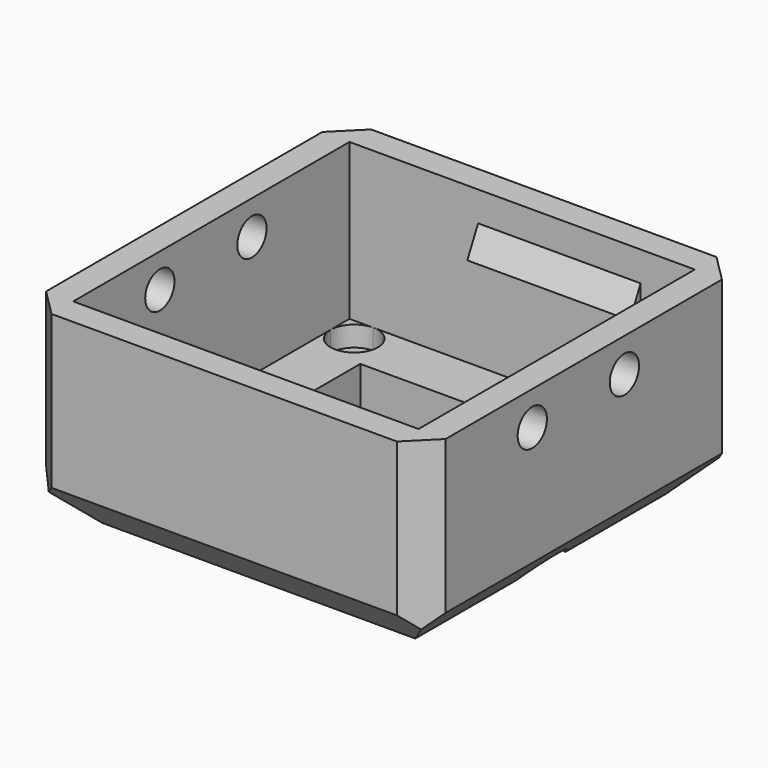
from build123d import *

# Parameters (mm, degrees)
F1_DEPTH     = 3
F0_W         = 29.5
F0_H         = 29.5
F2_DEPTH     = 14.5
F3_DEPTH     = 3
F4_DEPTH     = 1.5
F6_W         = 12
F6_H         = 2
F7_DEPTH     = 1
F8_SIZE2     = 1.99999
F8_SIZE      = 0.99999
F9_W         = 1.2
F9_H         = 2
F10_DEPTH    = 1
F11_SIZE2    = 1.99999
F11_SIZE     = 0.99999
F12_SIZE2    = 1.99999
F12_SIZE     = 0.99999
F13_T1_DEPTH = 45.958771123
F13_T3_DEPTH = 45.958771123
F5_R         = 1.35
F14_DEPTH    = 30
F15_SIZE     = 2


# Not quite as in the source:
# - a fillet or chamfer that OpenCascade refuses, or shapes differently, is made with other operations: its cross-section is extruded or revolved along the edge and cut away or added
# - a fillet or chamfer is up to 0.001 mm smaller than in the source, because OpenCascade refuses the exact size


with BuildPart() as f1:
    # F0 (on Top) → F1 (new body)
    with BuildSketch(Plane.XY):
        with BuildLine():
            ThreePointArc((12.75, 11), (9.7625631329, 9.7625631329), (11, 12.75))
            Line((11, 12.75), (-11, 12.75))
            ThreePointArc((-11, 12.75), (-9.7625631329, 12.2374368671), (-9.25, 11))
            ThreePointArc((-9.25, 11), (-11, 9.25), (-12.75, 11))
            Line((-12.75, 11), (-12.75, -5e-10))
            ThreePointArc((-12.75, -5e-10), (-11.9445436484, 1.9445436481), (-10, 2.75))
            Line((-10, 2.75), (-8.75, 2.75))
            Line((-8.75, 2.75), (-8.75, 8.75))
            Line((-8.75, 8.75), (8.75, 8.75))
            Line((8.75, 8.75), (8.75, 2.75))
            Line((8.75, 2.75), (10, 2.75))
            ThreePointArc((10, 2.75), (11.9445436484, 1.9445436481), (12.75, -5e-10))
            Line((12.75, -5e-10), (12.75, 11))
        make_face()
        with BuildLine():
            ThreePointArc((-12.75, 11), (-12.2374368671, 12.2374368671), (-11, 12.75))
            Line((-11, 12.75), (-12.75, 12.75))
            Line((-12.75, 12.75), (-12.75, 11))
        make_face()
        with BuildLine():
            Line((12.75, 11), (12.75, 12.75))
            Line((12.75, 12.75), (11, 12.75))
            ThreePointArc((11, 12.75), (12.2374368671, 12.2374368671), (12.75, 11))
        make_face()
        with BuildLine():
            ThreePointArc((12.75, 11), (12.2374368671, 12.2374368671), (11, 12.75))
            ThreePointArc((11, 12.75), (9.7625631329, 9.7625631329), (12.75, 11))
        make_face()
        with BuildLine():
            ThreePointArc((-9.25, 11), (-9.7625631329, 12.2374368671), (-11, 12.75))
            ThreePointArc((-11, 12.75), (-12.2374368671, 12.2374368671), (-12.75, 11))
            ThreePointArc((-12.75, 11), (-11, 9.25), (-9.25, 11))
        make_face()
    extrude(amount=F1_DEPTH)



with BuildPart() as f1b:
    # F0 (on Top) → F1, piece 2 (new body)
    with BuildSketch(Plane.XY):
        with BuildLine():
            Line((12.75, -11), (12.75, -5e-10))
            ThreePointArc((12.75, -5e-10), (11.9445436481, -1.9445436484), (10, -2.75))
            Line((10, -2.75), (8.75, -2.75))
            Line((8.75, -2.75), (8.75, -8.75))
            Line((8.75, -8.75), (-8.75, -8.75))
            Line((-8.75, -8.75), (-8.75, -2.75))
            Line((-8.75, -2.75), (-10, -2.75))
            ThreePointArc((-10, -2.75), (-11.9445436481, -1.9445436484), (-12.75, -5e-10))
            Line((-12.75, -5e-10), (-12.75, -11))
            ThreePointArc((-12.75, -11), (-11, -9.25), (-9.25, -11))
            ThreePointArc((-9.25, -11), (-9.7625631329, -12.2374368671), (-11, -12.75))
            Line((-11, -12.75), (11, -12.75))
            ThreePointArc((11, -12.75), (9.7625631329, -9.7625631329), (12.75, -11))
        make_face()
        with BuildLine():
            ThreePointArc((-11, -12.75), (-12.2374368671, -12.2374368671), (-12.75, -11))
            Line((-12.75, -11), (-12.75, -12.75))
            Line((-12.75, -12.75), (-11, -12.75))
        make_face()
        with BuildLine():
            Line((12.75, -12.75), (12.75, -11))
            ThreePointArc((12.75, -11), (12.2374368671, -12.2374368671), (11, -12.75))
            Line((11, -12.75), (12.75, -12.75))
        make_face()
        with BuildLine():
            ThreePointArc((11, -12.75), (12.2374368671, -12.2374368671), (12.75, -11))
            ThreePointArc((12.75, -11), (9.7625631329, -9.7625631329), (11, -12.75))
        make_face()
        with BuildLine():
            ThreePointArc((-9.25, -11), (-11, -9.25), (-12.75, -11))
            ThreePointArc((-12.75, -11), (-12.2374368671, -12.2374368671), (-11, -12.75))
            ThreePointArc((-11, -12.75), (-9.7625631329, -12.2374368671), (-9.25, -11))
        make_face()
    extrude(amount=F1_DEPTH)


with BuildPart() as f1_1:
    add(f1.part)

    add(f1b.part)  # F2 merges F1b
    # F0 (on Top) → F2 (join)
    with BuildSketch(Plane.XY):
        Rectangle(F0_W, F0_H)
        Polygon((11, 12.75), (12.75, 12.75), (12.75, 11), (12.75, -5e-10), (12.75, -11), (12.75, -12.75), (11, -12.75), (-11, -12.75), (-12.75, -12.75), (-12.75, -11), (-12.75, -5e-10), (-12.75, 11), (-12.75, 12.75), (-11, 12.75), align=None, mode=Mode.SUBTRACT)
    extrude(amount=F2_DEPTH)

    # F0 (on Top) → F3 (cut)
    with BuildSketch(Plane.XY):
        with BuildLine():
            ThreePointArc((-9.25, 11), (-9.7625631329, 12.2374368671), (-11, 12.75))
            ThreePointArc((-11, 12.75), (-12.2374368671, 12.2374368671), (-12.75, 11))
            ThreePointArc((-12.75, 11), (-11, 9.25), (-9.25, 11))
        make_face()
        with BuildLine():
            ThreePointArc((12.75, 11), (12.2374368671, 12.2374368671), (11, 12.75))
            ThreePointArc((11, 12.75), (9.7625631329, 9.7625631329), (12.75, 11))
        make_face()
        with BuildLine():
            ThreePointArc((-9.25, -11), (-11, -9.25), (-12.75, -11))
            ThreePointArc((-12.75, -11), (-12.2374368671, -12.2374368671), (-11, -12.75))
            ThreePointArc((-11, -12.75), (-9.7625631329, -12.2374368671), (-9.25, -11))
        make_face()
        with BuildLine():
            ThreePointArc((11, -12.75), (12.2374368671, -12.2374368671), (12.75, -11))
            ThreePointArc((12.75, -11), (9.7625631329, -9.7625631329), (11, -12.75))
        make_face()
    extrude(amount=F3_DEPTH, mode=Mode.SUBTRACT)

    # F0 (on Top) → F4 (join)
    with BuildSketch(Plane.XY):
        with BuildLine():
            ThreePointArc((12.75, 11), (12.2374368671, 12.2374368671), (11, 12.75))
            ThreePointArc((11, 12.75), (9.7625631329, 9.7625631329), (12.75, 11))
        make_face()
        with BuildLine():
            ThreePointArc((-9.25, 11), (-9.7625631329, 12.2374368671), (-11, 12.75))
            ThreePointArc((-11, 12.75), (-12.2374368671, 12.2374368671), (-12.75, 11))
            ThreePointArc((-12.75, 11), (-11, 9.25), (-9.25, 11))
        make_face()
        with BuildLine():
            ThreePointArc((-9.25, -11), (-11, -9.25), (-12.75, -11))
            ThreePointArc((-12.75, -11), (-12.2374368671, -12.2374368671), (-11, -12.75))
            ThreePointArc((-11, -12.75), (-9.7625631329, -12.2374368671), (-9.25, -11))
        make_face()
        with BuildLine():
            ThreePointArc((11, -12.75), (12.2374368671, -12.2374368671), (12.75, -11))
            ThreePointArc((12.75, -11), (9.7625631329, -9.7625631329), (11, -12.75))
        make_face()
    extrude(amount=F4_DEPTH)

    # F6 (on face) → F7 (join)
    with BuildSketch(Plane.XZ.offset(-12.75)):
        with Locations((2.75, 11.3)):
            Rectangle(F6_W, F6_H)
    extrude(amount=F7_DEPTH)

    # F8 (size 1 and 2 in the source; OpenCascade refuses exactly that, so slightly less here)
    f8_edges = [f1_1.edges().sort_by_distance(p)[0] for p in [
        (2.75, 11.75, 12.3),
    ]]
    f8_side = f1_1.faces().sort_by_distance((2.75, 12.25, 12.3))[0]
    chamfer(f8_edges, length=F8_SIZE, length2=F8_SIZE2, reference=f8_side)

    # F9 (on face) → F10 (join)
    with BuildSketch(Plane(origin=(0, -12.75, 0), x_dir=(-1, 0, 0), z_dir=(0, 1, 0))):
        with Locations((-8.85, 11.3)):
            Rectangle(F9_W, F9_H)
        with Locations((8.85, 11.3)):
            Rectangle(F9_W, F9_H)
    extrude(amount=F10_DEPTH)

    # F11 (size 1 and 2 in the source; OpenCascade refuses exactly that, so slightly less here)
    f11_edges = [f1_1.edges().sort_by_distance(p)[0] for p in [
        (8.85, -11.75, 12.3),
    ]]
    f11_side = f1_1.faces().sort_by_distance((8.85, -12.25, 12.3))[0]
    chamfer(f11_edges, length=F11_SIZE, length2=F11_SIZE2, reference=f11_side)

    # F12 (size 1 and 2 in the source; OpenCascade refuses exactly that, so slightly less here)
    f12_edges = [f1_1.edges().sort_by_distance(p)[0] for p in [
        (-8.85, -11.75, 12.3),
    ]]
    f12_side = f1_1.faces().sort_by_distance((-8.85, -12.25, 12.3))[0]
    chamfer(f12_edges, length=F12_SIZE, length2=F12_SIZE2, reference=f12_side)

    # F13: chamfer of 3.2 on 4 edges, made by hand

    # F13_s2 → F13_t1 (cut)
    with BuildSketch(Plane.YZ.offset(-22.9793855615)):
        Polygon((14.75, 3.2), (11.55, 0), (14.75, 0), align=None)
        Polygon((-14.75, 3.2), (-11.55, 0), (-14.75, 0), align=None)
    extrude(amount=F13_T1_DEPTH, mode=Mode.SUBTRACT)

    # F13_s4 → F13_t3 (cut)
    with BuildSketch(Plane.XZ.offset(-22.9793855615)):
        Polygon((-14.75, 3.2), (-11.55, 0), (-14.75, 0), align=None)
        Polygon((14.75, 3.2), (11.55, 0), (14.75, 0), align=None)
    extrude(amount=F13_T3_DEPTH, mode=Mode.SUBTRACT)

    # F5 (on face) → F14 (cut)
    with BuildSketch(Plane(origin=(-14.75, 0, 0), x_dir=(0, -1, 0), z_dir=(-1, 0, 0))):
        with Locations((4.75, 12)):
            Circle(F5_R)
        with Locations((-3.75, 12)):
            Circle(F5_R)
    extrude(amount=-F14_DEPTH, mode=Mode.SUBTRACT)

    # F15
    f15_edges = [f1_1.edges().sort_by_distance(p)[0] for p in [
        (14.75, 14.75, 8.85),
        (-14.75, 14.75, 8.85),
        (14.75, -14.75, 8.85),
        (-14.75, -14.75, 8.85),
    ]]
    chamfer(f15_edges, length=F15_SIZE)


solid = f1_1.part
